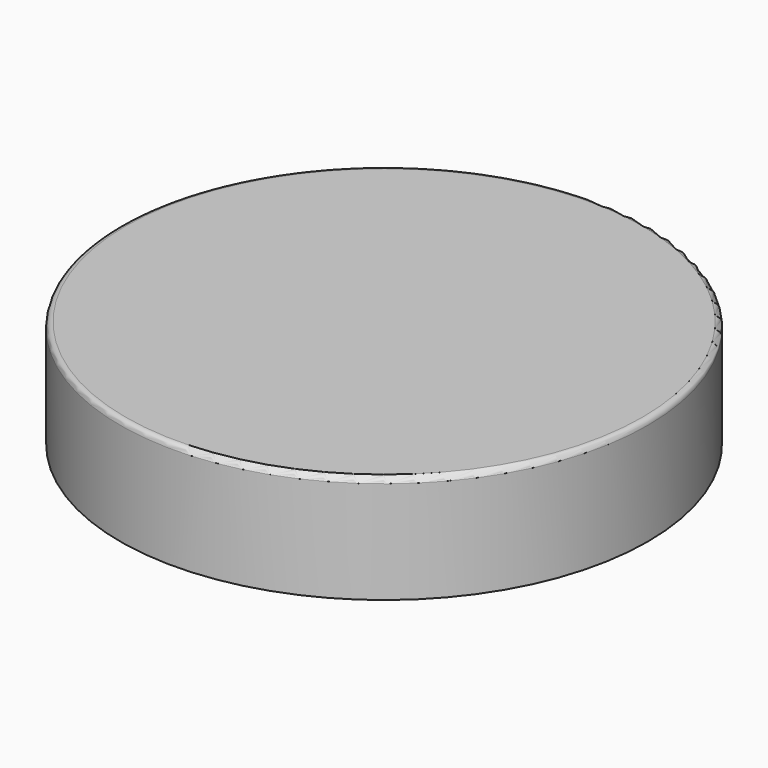
from build123d import *

# Parameters (mm, degrees)
F0_R     = 9.8
F0_R_2   = 9.65
F1_DEPTH = 4
F2_DEPTH = 3
F3_R     = 0.2


with BuildPart() as f1:
    # F0 (on Top) → F1 (new body)
    with BuildSketch(Plane.XY):
        Circle(F0_R)
        Circle(F0_R_2, mode=Mode.SUBTRACT)
        Circle(F0_R_2)
    extrude(amount=F1_DEPTH)

    # F0 (on Top) → F2 (cut)
    with BuildSketch(Plane.XY):
        Circle(F0_R_2)
    extrude(amount=F2_DEPTH, mode=Mode.SUBTRACT)

    # F3
    f3_edges = [f1.edges().sort_by_distance(p)[0] for p in [
        (-9.8, 0, 4),
        (-9.65, 0, 3),
    ]]
    fillet(f3_edges, radius=F3_R)


solid = f1.part
